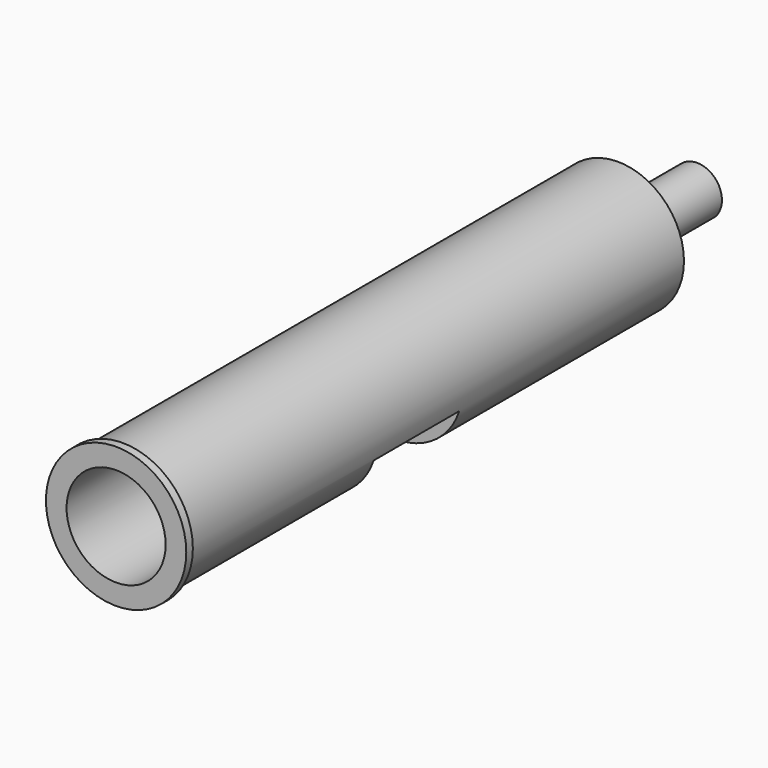
from build123d import *

# Parameters (mm, degrees)
F0_R     = 4
F0_R_2   = 3
F1_DEPTH = 38
F2_R     = 4.25
F2_R_2   = 4
F2_R_3   = 3
F3_DEPTH = 0.5
F4_W     = 6.49
F4_H     = 2.75
F5_DEPTH = 12.5
F6_R     = 4
F6_R_2   = 3
F7_DEPTH = 2.5
F9_DEPTH = 6


with BuildPart() as f1:
    # F0 (on Front) → F1 (new body)
    with BuildSketch(Plane.XZ):
        Circle(F0_R)
        Circle(F0_R_2, mode=Mode.SUBTRACT)
    extrude(amount=-F1_DEPTH)

    # F2 (on face) → F3 (join)
    with BuildSketch(Plane.XZ):
        Circle(F2_R)
        Circle(F2_R_2, mode=Mode.SUBTRACT)
        Circle(F2_R_2)
        Circle(F2_R_3, mode=Mode.SUBTRACT)
    extrude(amount=-F3_DEPTH)

    # F4 (on Right) → F5 (cut, symmetric)
    with BuildSketch(Plane.YZ):
        with Locations((17.995, -2.625)):
            Rectangle(F4_W, F4_H)
    extrude(amount=F5_DEPTH, both=True, mode=Mode.SUBTRACT)

    # F6 (on face) → F7 (join)
    with BuildSketch(Plane(origin=(0, 38, 0), x_dir=(-1, 0, 0), z_dir=(0, 1, 0))):
        Circle(F6_R)
        Circle(F6_R_2, mode=Mode.SUBTRACT)
        Circle(F6_R_2)
    extrude(amount=-F7_DEPTH)

    # F8 (on face) → F9 (join)
    with BuildSketch(Plane(origin=(0, 38, 0), x_dir=(-1, 0, 0), z_dir=(0, 1, 0))):
        with BuildLine():
            Line((-1.1180339887, -1), (1.1180339887, -1))
            ThreePointArc((1.1180339887, -1), (0, 1.5), (-1.1180339887, -1))
        make_face()
    extrude(amount=F9_DEPTH)


solid = f1.part
